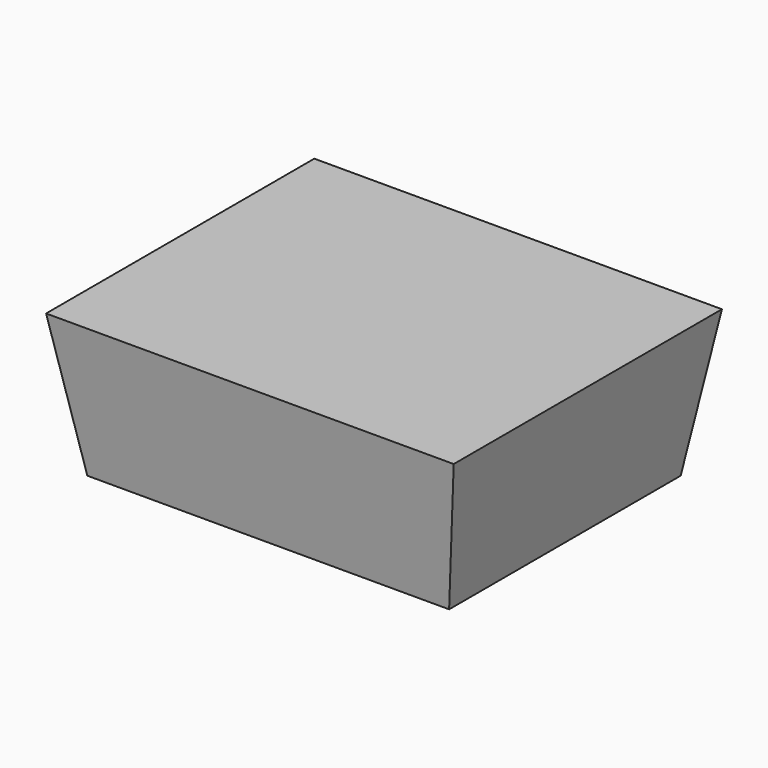
from build123d import *

# Parameters (mm, degrees)
F0_W     = 250
F0_H     = 200
F1_DEPTH = 100
F1_TAPER = -9


# Not quite as in the source:
# - the program builds the solid bodies; features that only make, move or delete a surface that nothing else refers to are left out


with BuildPart() as f1:
    # F0 (on Top) → F1 (new body)
    with BuildSketch(Plane.XY):
        Rectangle(F0_W, F0_H)
    extrude(amount=F1_DEPTH, taper=F1_TAPER)


solid = f1.part
